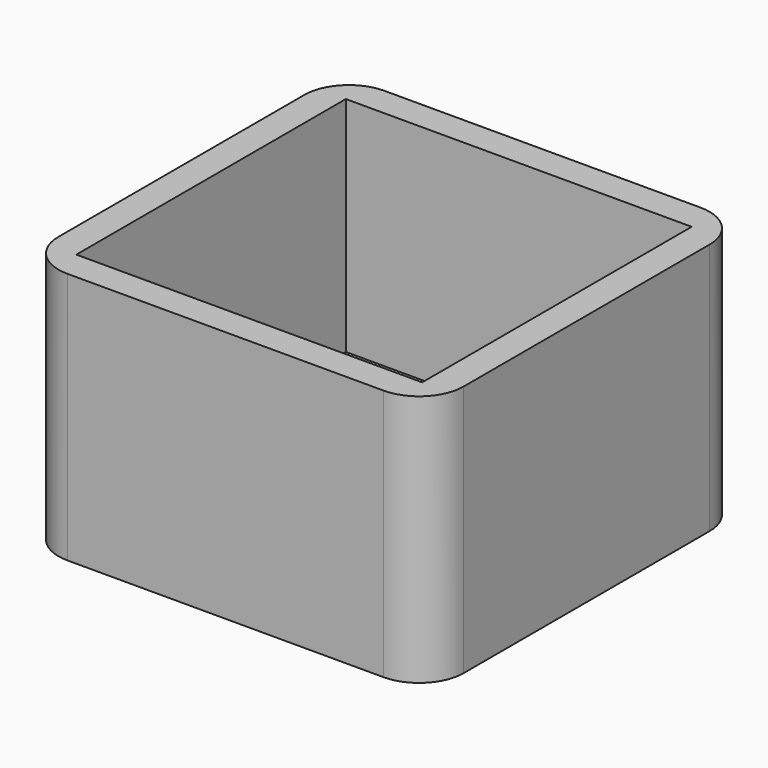
from build123d import *

# Parameters (mm, degrees)
F0_W        = 23.3
F0_H        = 22.7
F1_DEPTH    = 15
F2_T        = 2
F3_T1_DEPTH = 32
F5_DEPTH    = 25


# Not quite as in the source:
# - a fillet or chamfer that OpenCascade refuses, or shapes differently, is made with other operations: its cross-section is extruded or revolved along the edge and cut away or added


with BuildPart() as f1:
    # F0 (on Top) → F1 (new body)
    with BuildSketch(Plane.XY):
        with Locations((-11.65, 11.35)):
            Rectangle(F0_W, F0_H)
    extrude(amount=F1_DEPTH)

    # F2
    f2_openings = [f1.faces().sort_by_distance(p)[0] for p in [
        (-11.65, 11.35, 15),
    ]]
    offset(amount=F2_T, openings=f2_openings, kind=Kind.INTERSECTION)

    # F3: fillet of radius 3 on 4 edges, made by hand

    # F3_s2 → F3_t1 (cut)
    with BuildSketch(Plane.XY.offset(-9.5)):
        with BuildLine():
            ThreePointArc((-22.3, -2), (-24.4213203436, -1.1213203436), (-25.3, 1))
            Line((-25.3, 1), (-25.3, -2))
            Line((-25.3, -2), (-22.3, -2))
        make_face()
        with BuildLine():
            ThreePointArc((-1, -2), (1.1213203436, -1.1213203436), (2, 1))
            Line((2, 1), (2, -2))
            Line((2, -2), (-1, -2))
        make_face()
        with BuildLine():
            ThreePointArc((2, 21.7), (1.1213203436, 23.8213203436), (-1, 24.7))
            Line((-1, 24.7), (2, 24.7))
            Line((2, 24.7), (2, 21.7))
        make_face()
        with BuildLine():
            ThreePointArc((-22.3, 24.7), (-24.4213203436, 23.8213203436), (-25.3, 21.7))
            Line((-25.3, 21.7), (-25.3, 24.7))
            Line((-25.3, 24.7), (-22.3, 24.7))
        make_face()
    extrude(amount=F3_T1_DEPTH, mode=Mode.SUBTRACT)

    # F4 (on face) → F5 (cut)
    with BuildSketch(Plane(origin=(0, 0, -2), x_dir=(1, 0, 0), z_dir=(0, 0, -1))):
        Polygon((-18.8904213403, -15.5302592099), (-11.65, -19.7105184197), (-4.4095786597, -15.5302592099), (-4.4095786597, -7.1697407901), (-11.65, -2.9894815803), (-18.8904213403, -7.1697407901), align=None)
    extrude(amount=-F5_DEPTH, mode=Mode.SUBTRACT)


solid = f1.part
